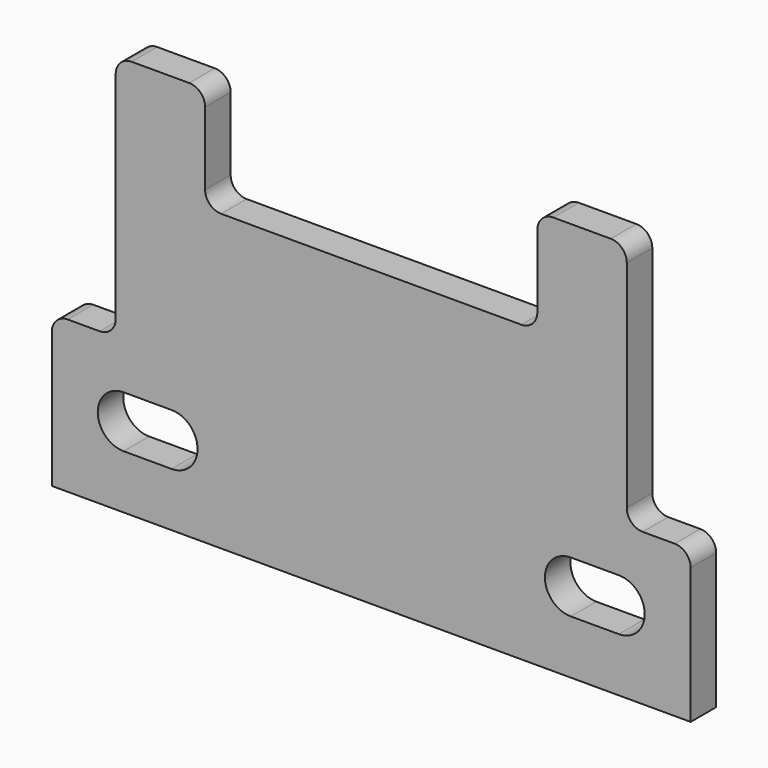
from build123d import *

# Parameters (mm, degrees)
F1_DEPTH = 3.175
F2_R     = 1.5875
F4_DEPTH = 3.175


with BuildPart() as f1:
    # F0 (on Front) → F1 (new body)
    with BuildSketch(Plane.XZ):
        Polygon((0, 15.08125), (0, 0), (63.5, 0), (63.5, 15.08125), (57.15, 15.08125), (57.15, 39.7002), (48.26, 39.7002), (48.26, 29.2862), (15.24, 29.2862), (15.24, 39.7002), (6.35, 39.7002), (6.35, 15.08125), align=None)
    extrude(amount=F1_DEPTH)

    # F2
    f2_edges = [f1.edges().sort_by_distance(p)[0] for p in [
        (6.35, -1.5875, 39.7002),
        (6.35, -1.5875, 15.08125),
        (0, -1.5875, 15.08125),
        (15.24, -1.5875, 39.7002),
        (48.26, -1.5875, 39.7002),
        (57.15, -1.5875, 39.7002),
        (57.15, -1.5875, 15.08125),
        (63.5, -1.5875, 15.08125),
        (48.26, -1.5875, 29.2862),
        (15.24, -1.5875, 29.2862),
    ]]
    fillet(f2_edges, radius=F2_R)

    # F3 (on face) → F4 (cut)
    with BuildSketch(Plane.XZ.offset(3.175)):
        with BuildLine():
            Line((51.59375, 5.3594), (56.35625, 5.3594))
            ThreePointArc((56.35625, 5.3594), (58.93435, 7.9375), (56.35625, 10.5156))
            Line((56.35625, 10.5156), (51.59375, 10.5156))
            ThreePointArc((51.59375, 10.5156), (49.01565, 7.9375), (51.59375, 5.3594))
        make_face()
        with BuildLine():
            Line((7.14375, 5.3594), (11.90625, 5.3594))
            ThreePointArc((11.90625, 5.3594), (14.48435, 7.9375), (11.90625, 10.5156))
            Line((11.90625, 10.5156), (7.14375, 10.5156))
            ThreePointArc((7.14375, 10.5156), (4.56565, 7.9375), (7.14375, 5.3594))
        make_face()
    extrude(amount=-F4_DEPTH, mode=Mode.SUBTRACT)


solid = f1.part
